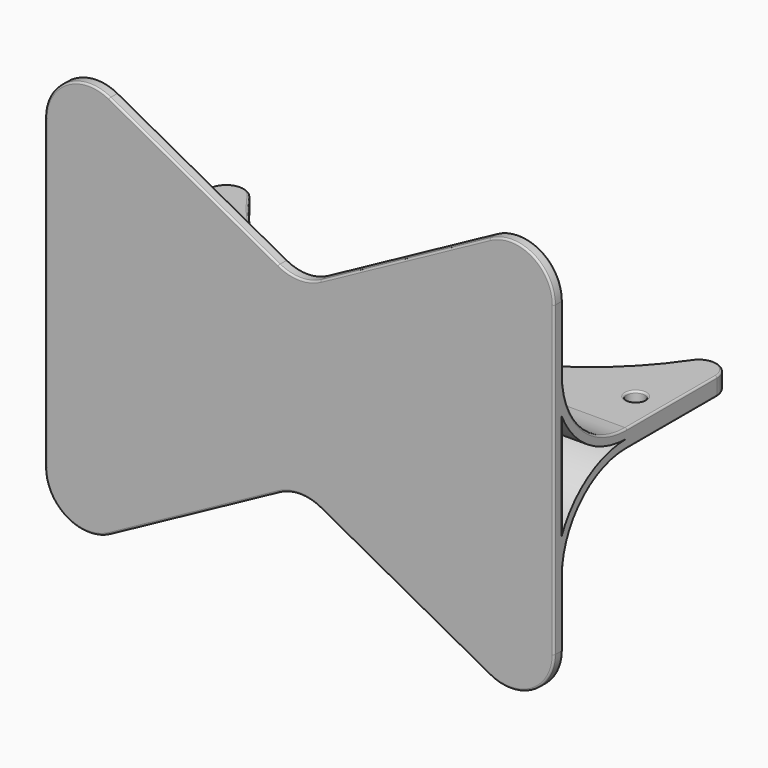
from build123d import *

# Parameters (mm, degrees)
F0_R     = 2.5
F1_DEPTH = 5
F3_DEPTH = 140
F4_DEPTH = 140.001
F5_F1_R  = 5
F5_F2_R  = 5
F7_DEPTH = 3.001
F8_R     = 12
F9_R     = 0.5


# Not quite as in the source:
# - a feature names something its author has since deleted; it is built from what else it names


with BuildPart() as f1:
    # F0 (on Top) → F1 (new body)
    with BuildSketch(Plane.XY):
        with BuildLine():
            ThreePointArc((70, -22.410934831), (0, -73.5), (-70, -22.410934831))
            Line((-70, -22.410934831), (-70, -75))
            Line((-70, -75), (70, -75))
            Line((70, -75), (70, -22.410934831))
        make_face()
        with Locations((-62.25, -62.25)):
            Circle(F0_R, mode=Mode.SUBTRACT)
        with Locations((62.25, -62.25)):
            Circle(F0_R, mode=Mode.SUBTRACT)
    extrude(amount=F1_DEPTH)

    # F2 (on face) → F3 (join, through all)
    with BuildSketch(Plane(origin=(-70, 0, 0), x_dir=(0, -1, 0), z_dir=(-1, 0, 0))):
        with BuildLine():
            ThreePointArc((75, 0), (90.5563491861, -6.4436508139), (97, -22))
            Line((97, -22), (97, -60))
            Line((97, -60), (100, -60))
            Line((100, -60), (100, 65))
            Line((100, 65), (97, 65))
            Line((97, 65), (97, 27))
            ThreePointArc((97, 27), (90.5563491861, 11.4436508139), (75, 5))
            Line((75, 5), (75, 2.5))
            Line((75, 2.5), (75, 0))
        make_face()
        with BuildLine():
            ThreePointArc((97, -11.2180706736), (87.9632698711, -1.2104922076), (75, 2.5))
            ThreePointArc((75, 2.5), (87.9632698711, 6.2104922076), (97, 16.2180706736))
            Line((97, 16.2180706736), (97, -11.2180706736))
        make_face(mode=Mode.SUBTRACT)
        with BuildLine():
            ThreePointArc((97, 16.2180706736), (87.9632698711, 6.2104922076), (75, 2.5))
            ThreePointArc((75, 2.5), (87.9632698711, -1.2104922076), (97, -11.2180706736))
            Line((97, -11.2180706736), (97, 16.2180706736))
        make_face()
    extrude(amount=-F3_DEPTH)

    # F2 (on face) → F4 (cut, through all)
    with BuildSketch(Plane(origin=(-70, 0, 0), x_dir=(0, -1, 0), z_dir=(-1, 0, 0))):
        with BuildLine():
            ThreePointArc((97, 16.2180706736), (87.9632698711, 6.2104922076), (75, 2.5))
            ThreePointArc((75, 2.5), (87.9632698711, -1.2104922076), (97, -11.2180706736))
            Line((97, -11.2180706736), (97, 16.2180706736))
        make_face()
    extrude(amount=-F4_DEPTH, mode=Mode.SUBTRACT)

    # F5: fillet of radius 5 on 2 edges, made by hand

    # F5_f1
    f5_f1_edges = [f1.edges().sort_by_distance(p)[0] for p in [
        (70, -22.410934831, 2.5),
    ]]
    fillet(f5_f1_edges, radius=F5_F1_R)

    # F5_f2
    f5_f2_edges = [f1.edges().sort_by_distance(p)[0] for p in [
        (-70, -22.410934831, 2.5),
    ]]
    fillet(f5_f2_edges, radius=F5_F2_R)

    # F6 (on face) → F7 (cut, through all)
    with BuildSketch(Plane(origin=(0, -97, 0), x_dir=(-1, 0, 0), z_dir=(0, 1, 0))):
        Polygon((0, 27), (70, 65), (0, 65), (-70, 65), align=None)
        Polygon((0, -60), (70, -60), (0, -22), (-70, -60), align=None)
    extrude(amount=-F7_DEPTH, mode=Mode.SUBTRACT)

    # F8
    f8_edges = [f1.edges().sort_by_distance(p)[0] for p in [
        (0, -98.5, 27),
        (-70, -98.5, 65),
        (70, -98.5, 65),
        (0, -98.5, -22),
        (-70, -98.5, -60),
        (70, -98.5, -60),
    ]]
    fillet(f8_edges, radius=F8_R)

    # F9
    f9_edges = [f1.edges().sort_by_distance(p)[0] for p in [
        (0, -73.5, 0),
        (-70, -97, 2.5),
        (-35, -97, 27),
        (35, -97, 27),
        (0, -75, 5),
        (-70, -90.556349, 11.443651),
        (70, -90.556349, 11.443651),
        (-70, -97, 35.91578),
        (-64.13591, -97, 55.144204),
        (-29, -97, 42.742857),
        (-2.862551, -97, 28.553956),
        (29, -97, 42.742857),
        (64.13591, -97, 55.144204),
        (0, -97, 28.654154),
        (70, -97, 35.91578),
        (70, -97, 2.5),
        (70, -100, 2.5),
        (-70, -100, 2.5),
        (64.75, -62.25, 2.5),
        (59.75, -62.25, 0),
        (59.75, -62.25, 5),
        (-59.75, -62.25, 2.5),
        (-64.75, -62.25, 0),
        (-64.75, -62.25, 5),
        (-70, -97, -30.91578),
        (-70, -90.556349, -6.443651),
        (-70, -59.507101, 0),
        (-70, -59.507101, 5),
        (-64.13591, -97, -50.144204),
        (-29, -97, -37.742857),
        (-64.13591, -100, -50.144204),
        (70, -90.556349, -6.443651),
        (-64.13591, -100, 55.144204),
        (-29, -100, -37.742857),
        (-29, -100, 42.742857),
        (0, -100, -23.654154),
        (0, -100, 28.654154),
        (29, -100, -37.742857),
        (29, -100, 42.742857),
        (64.13591, -100, -50.144204),
        (64.13591, -100, 55.144204),
        (-66.466179, -39.234002, 0),
        (66.466179, -39.234002, 0),
        (70, -59.507101, 0),
        (-66.466179, -39.234002, 5),
        (0, -73.5, 5),
        (66.466179, -39.234002, 5),
        (70, -59.507101, 5),
        (29, -97, -37.742857),
        (0, -97, -23.654154),
        (64.13591, -97, -50.144204),
        (70, -97, -30.91578),
    ]]
    fillet(f9_edges, radius=F9_R)


solid = f1.part
